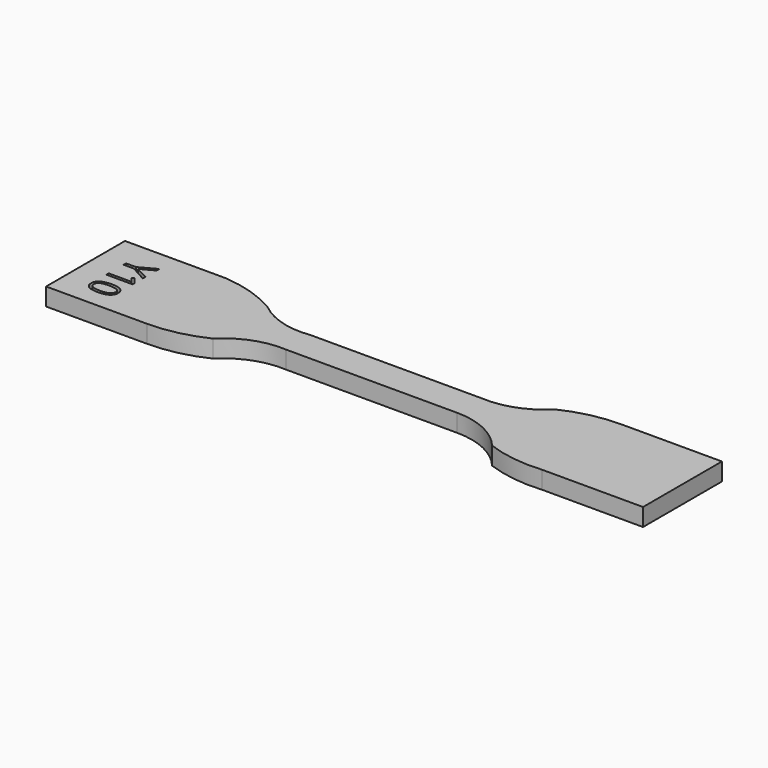
from build123d import *

# Parameters (mm, degrees)
F1_DEPTH     = 3.4
F2_TEXT_SIZE = 7.0564552314
F3_DEPTH     = 1


# Not quite as in the source:
# - Text() gives the source's letters only with a copy of the font that has no kerning and outlines rounded to 1/6400 em; it was checked with that copy


with BuildPart() as f1:
    # F0 (on Top) → F1 (new body)
    with BuildSketch(Plane.XY):
        with BuildLine():
            Line((-14.4320548165, 19.7811394548), (-33.8720548165, 19.7811394548))
            Line((-33.8720548165, 19.7811394548), (-33.8720548165, 0.7811394548))
            Line((-33.8720548165, 0.7811394548), (-14.4320548165, 0.7811394548))
            ThreePointArc((-14.4320548165, 0.7811394548), (-8.9053122052, 1.3996892086), (-3.6520548165, 3.2247301661))
            ThreePointArc((-3.6520548165, 3.2247301661), (1.3014698263, 6.4128780055), (7.1279451835, 7.2811394548))
            Line((7.1279451835, 7.2811394548), (40.1279451835, 7.2811394548))
            ThreePointArc((40.1279451835, 7.2811394548), (46.0837574042, 5.9511158081), (50.9079451835, 2.2137538538))
            ThreePointArc((50.9079451835, 2.2137538538), (56.2191047011, 0.9041953221), (61.6879451835, 0.7811394548))
            Line((61.6879451835, 0.7811394548), (81.1279451835, 0.7811394548))
            Line((81.1279451835, 0.7811394548), (81.1279451835, 19.7811394548))
            Line((81.1279451835, 19.7811394548), (61.6879451835, 19.7811394548))
            ThreePointArc((61.6879451835, 19.7811394548), (56.1612025723, 19.162589701), (50.9079451835, 17.3375487435))
            ThreePointArc((50.9079451835, 17.3375487435), (45.9544205407, 14.1494009041), (40.1279451835, 13.2811394548))
            Line((40.1279451835, 13.2811394548), (7.1279451835, 13.2811394548))
            ThreePointArc((7.1279451835, 13.2811394548), (1.4167452884, 13.6925537245), (-3.6520548165, 16.3560723447))
            ThreePointArc((-3.6520548165, 16.3560723447), (-8.8458057958, 18.686276846), (-14.4320548165, 19.7811394548))
        make_face()
    extrude(amount=F1_DEPTH)

    # F2 (on face) → F3 (cut)
    with BuildSketch(Plane.XY.offset(3.4)):
        with Locations(Location((-29.1824135929, 15.8650862949), (0, 0, -90))):
            Text('Y10', F2_TEXT_SIZE, font='Open Sans', text_align=(TextAlign.LEFT, TextAlign.BOTTOM))
    extrude(amount=-F3_DEPTH, mode=Mode.SUBTRACT)


solid = f1.part
